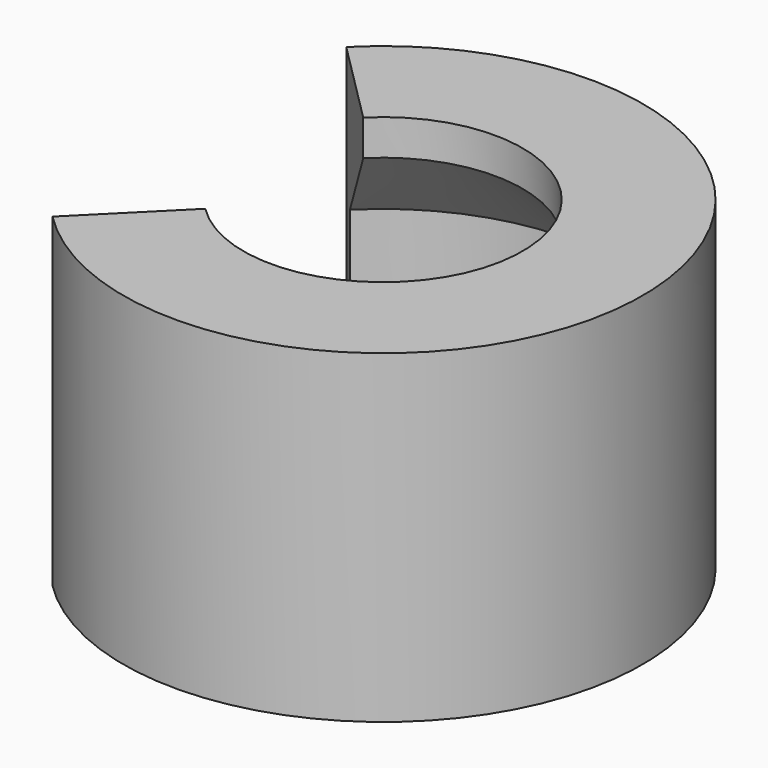
from build123d import *

# Parameters (mm, degrees)
F1_ANGLE_BACK = 135
F1_ANGLE      = 270
F2_SIZE       = 0.4
F3_SIZE       = 1.44999


# Not quite as in the source:
# - a fillet or chamfer is up to 0.001 mm smaller than in the source, because OpenCascade refuses the exact size


with BuildPart() as f1:
    # F0 (on Front) → F1 (revolve)
    with BuildSketch(Plane.XZ, mode=Mode.PRIVATE) as f1_sk:
        Polygon((2.65, 1.5), (2.65, 0), (4, 0), (4, 5), (2.15, 5), (2.15, 3), (3.6, 3), (3.6, 1.5), align=None)
    revolve(f1_sk.sketch.rotate(Axis((0, 0, 2.5), (0, 0, -1)), -F1_ANGLE_BACK), axis=Axis((0, 0, 2.5), (0, 0, -1)), revolution_arc=F1_ANGLE)

    # F2
    f2_edges = [f1.edges().sort_by_distance(p)[0] for p in [
        (2.65, 0, 1.5),
    ]]
    chamfer(f2_edges, length=F2_SIZE)

    # F3 (size 1.45 in the source; OpenCascade refuses exactly that, so slightly less here)
    f3_edges = [f1.edges().sort_by_distance(p)[0] for p in [
        (2.15, 0, 3),
    ]]
    chamfer(f3_edges, length=F3_SIZE)


solid = f1.part
